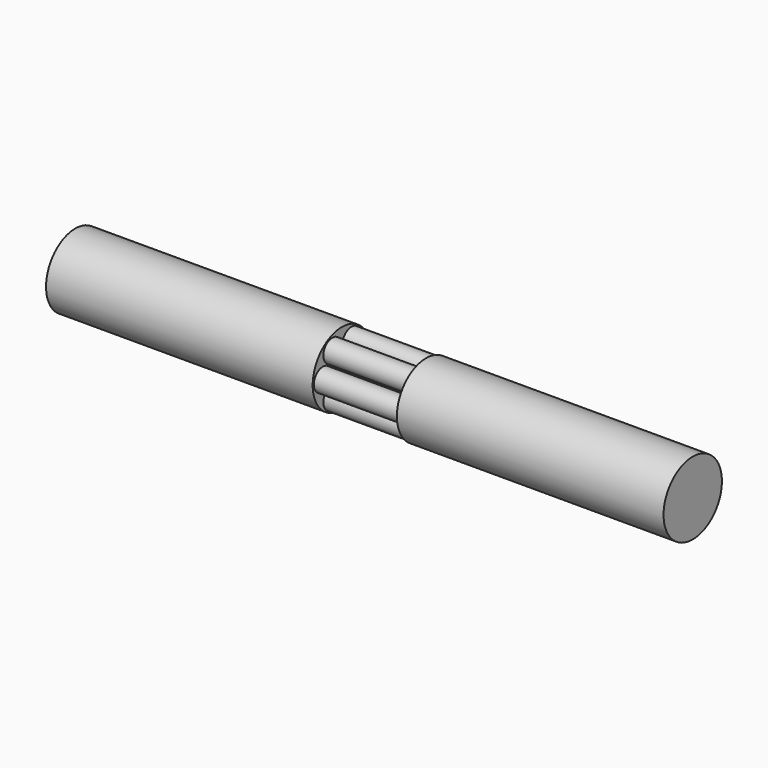
from build123d import *

# Parameters (mm, degrees)
F0_R     = 26
F1_DEPTH = 220
F2_R     = 8
F3_DEPTH = 50
F4_COUNT = 6
F6_D     = 15.98
F6_DEPTH = 50
F6_TIP   = 4.800876346
F5_R     = 26
F5_R_2   = 14.7224318643
F7_DEPTH = 30


with BuildPart() as f1:
    # F0 (on Right) → F1 (new body)
    with BuildSketch(Plane.YZ):
        Circle(F0_R)
    extrude(amount=-F1_DEPTH)

    # F6
    with Locations(Plane.YZ):
        with Locations((-8.5, 14.7224318643), (8.5, 14.7224318643), (-17, 0), (-8.5, -14.7224318643), (8.5, -14.7224318643), (17, 0)):
            Hole(F6_D / 2, depth=F6_DEPTH)
            with Locations((0, 0, -(F6_DEPTH + F6_TIP / 2))):  # 118° drill point
                Cone(0, F6_D / 2, F6_TIP, mode=Mode.SUBTRACT)

    # F5 (on Right) → F7 (cut)
    with BuildSketch(Plane.YZ):
        Circle(F5_R)
        Circle(F5_R_2, mode=Mode.SUBTRACT)
    extrude(amount=-F7_DEPTH, mode=Mode.SUBTRACT)


with BuildPart() as f3:
    # F2 (on Right) → F3 (new body, symmetric)
    with BuildSketch(Plane.YZ):
        with Locations((8.5, -14.7224318643)):
            Circle(F2_R)
    extrude(amount=F3_DEPTH, both=True)


with BuildPart() as f4_1:
    # F4: instance of F3
    add(f3.part.rotate(Axis((0, 0, 0), (1, 0, 0)), 1 * 360 / F4_COUNT))


with BuildPart() as f4_2:
    # F4: instance of F3
    add(f3.part.rotate(Axis((0, 0, 0), (1, 0, 0)), 2 * 360 / F4_COUNT))


with BuildPart() as f4_3:
    # F4: instance of F3
    add(f3.part.rotate(Axis((0, 0, 0), (1, 0, 0)), 3 * 360 / F4_COUNT))


with BuildPart() as f4_4:
    # F4: instance of F3
    add(f3.part.rotate(Axis((0, 0, 0), (1, 0, 0)), 4 * 360 / F4_COUNT))


with BuildPart() as f4_5:
    # F4: instance of F3
    add(f3.part.rotate(Axis((0, 0, 0), (1, 0, 0)), 5 * 360 / F4_COUNT))


with BuildPart() as f8_1:
    # F8: instance of F1
    add(f1.part.mirror(Plane.YZ))


solid = Compound([f1.part, f3.part, f4_1.part, f4_2.part, f4_3.part, f4_4.part, f4_5.part, f8_1.part])
